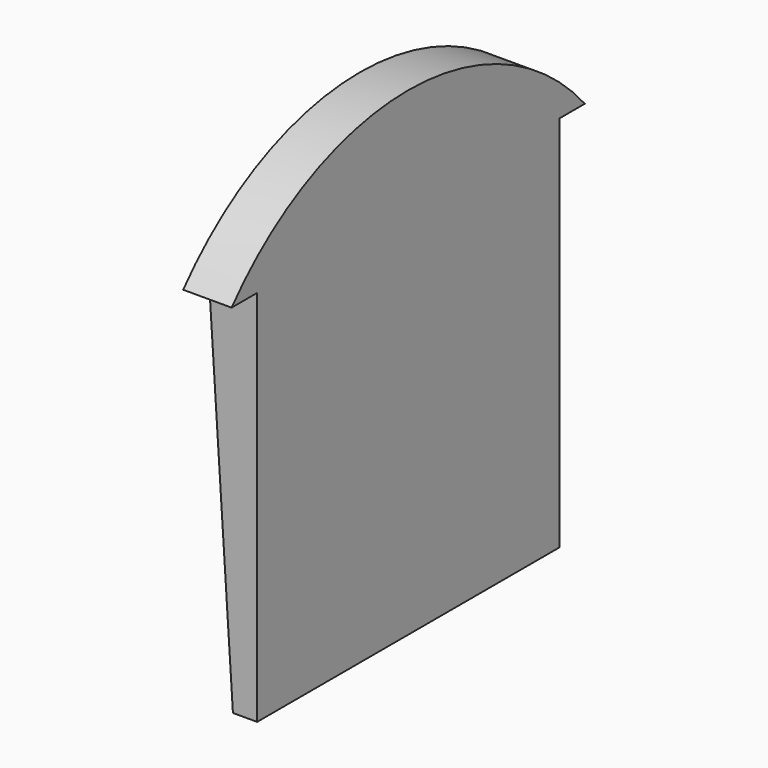
from build123d import *

# Parameters (mm, degrees)
F0_W     = 7.8
F0_H     = 7.8
F1_DEPTH = 1
F2_SIZE2 = 0.5
F2_SIZE  = 7.8


# Not quite as in the source:
# - a feature names something its author has since deleted; it is built from what else it names


with BuildPart() as f1:
    # F0 (on Right) → F1 (new body)
    with BuildSketch(Plane.YZ):
        with BuildLine():
            Line((-3.9, 1.419822283), (3.9, 1.419822283))
            Line((3.9, 1.419822283), (4.5596052461, 1.419822283))
            ThreePointArc((4.5596052461, 1.419822283), (0, 3.519822283), (-4.5596052461, 1.419822283))
            Line((-4.5596052461, 1.419822283), (-3.9, 1.419822283))
        make_face()
        with Locations((0, -2.480177717)):
            Rectangle(F0_W, F0_H)
    extrude(amount=F1_DEPTH)

    # F2
    f2_edges = [f1.edges().sort_by_distance(p)[0] for p in [
        (0, 0, -6.380178),
    ]]
    f2_side = f1.faces().sort_by_distance((0, 0, -1.62771))[0]
    chamfer(f2_edges, length=F2_SIZE, length2=F2_SIZE2, reference=f2_side)


solid = f1.part
